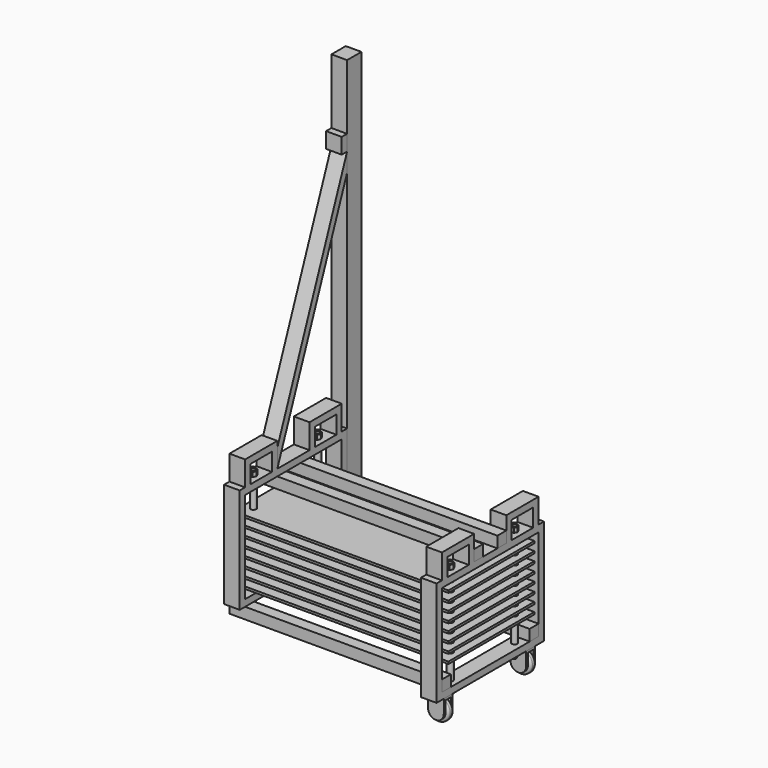
from build123d import *

# Parameters (mm, degrees)
F0_W           = 1219.2
F0_H           = 609.6
F0_R           = 12.7
F1_DEPTH       = 12.7
F9_R           = 15.875
F9_R_2         = 12.7
F10_DEPTH      = 127
F10_DEPTH_BACK = 393.7
F29_DEPTH      = 25.4
F29_DEPTH_BACK = 495.3
F9_R_3         = 9.525
F46_DEPTH      = 203.2
F46_DEPTH_BACK = 469.9
F47_DEPTH      = 101.6
F47_DEPTH_BACK = 571.5
F49_DEPTH      = 88.9
F57_W          = 38.1
F57_H          = 520.7
F58_DEPTH      = 88.9
F59_W          = 38.1
F59_H          = 520.7
F60_DEPTH      = 88.9
F62_DEPTH      = 88.9
F64_DEPTH      = 88.9
F66_DEPTH      = 710.8932972611
F67_R          = 60.325
F68_DEPTH      = 38.1
F69_R          = 12.7
F71_R          = 9.525
F72_DEPTH      = 25.4
F84_DEPTH      = 88.9
F85_W          = 63.5
F85_H          = 63.5
F86_DEPTH      = 1206.5
F88_DEPTH      = 88.9
F90_DEPTH      = 88.9
F89_W          = 38.1
F89_H          = 88.9
F91_DEPTH      = 88.9


with BuildPart() as f1:
    # F0 (on Top) → F1 (new body)
    with BuildSketch(Plane.XY):
        with Locations((1.1357478797, 12.4982790879)):
            Rectangle(F0_W, F0_H)
        with Locations((-557.6642521203, -216.1017209121)):
            Circle(F0_R, mode=Mode.SUBTRACT)
        with Locations((559.9357478797, -216.1017209121)):
            Circle(F0_R, mode=Mode.SUBTRACT)
        with Locations((-557.6642521203, 241.0982790879)):
            Circle(F0_R, mode=Mode.SUBTRACT)
        with Locations((559.9357478797, 241.0982790879)):
            Circle(F0_R, mode=Mode.SUBTRACT)
    extrude(amount=F1_DEPTH)


with BuildPart() as f2_1:
    # F2: copy of F1
    add(f1.part.moved(Location((0, 0, -50.8))))


with BuildPart() as f3_1:
    # F3: copy of F2_1
    add(f2_1.part.moved(Location((0, 0, -50.8))))


with BuildPart() as f4_1:
    # F4: copy of F3_1
    add(f3_1.part.moved(Location((0, 0, -50.8))))


with BuildPart() as f5_1:
    # F5: copy of F4_1
    add(f4_1.part.moved(Location((0, 0, -50.8))))


with BuildPart() as f6_1:
    # F6: copy of F5_1
    add(f5_1.part.moved(Location((0, 0, -50.8))))


with BuildPart() as f7_1:
    # F7: copy of F6_1
    add(f6_1.part.moved(Location((0, 0, -50.8))))


with BuildPart() as f8_1:
    # F8: copy of F7_1
    add(f7_1.part.moved(Location((0, 0, -50.8))))


with BuildPart() as f10:
    # F9 (on face) → F10 (new body, two sides)
    with BuildSketch(Plane.XY.offset(12.7)) as f10_sk:
        with Locations((-557.6642521203, 241.0982790879)):
            Circle(F9_R)
        with Locations((-557.6642521203, 241.0982790879)):
            Circle(F9_R_2, mode=Mode.SUBTRACT)
    extrude(amount=F10_DEPTH)
    extrude(f10_sk.sketch, amount=-F10_DEPTH_BACK)

    # F12: cut F1
    add(f1.part, mode=Mode.SUBTRACT)

    # F14: cut F2_1
    add(f2_1.part, mode=Mode.SUBTRACT)


with BuildPart() as f10b:
    # F9 (on face) → F10, piece 2 (new body, two sides)
    with BuildSketch(Plane.XY.offset(12.7)) as f10_2_sk:
        with Locations((-557.6642521203, -216.1017209121)):
            Circle(F9_R)
        with Locations((-557.6642521203, -216.1017209121)):
            Circle(F9_R_2, mode=Mode.SUBTRACT)
    extrude(amount=F10_DEPTH)
    extrude(f10_2_sk.sketch, amount=-F10_DEPTH_BACK)

    # F12: cut F1
    add(f1.part, mode=Mode.SUBTRACT)

    # F14: cut F2_1
    add(f2_1.part, mode=Mode.SUBTRACT)


with BuildPart() as f11_1:
    # F11: copy of F1
    add(f1.part)


with BuildPart() as f13_1:
    # F13: copy of F2_1
    add(f2_1.part)


with BuildPart() as f15_1:
    # F15: copy of F13_1
    add(f13_1.part)


with BuildPart() as f10_1:
    add(f10.part)

    # F16: cut F13_1
    add(f13_1.part, mode=Mode.SUBTRACT)


with BuildPart() as f10b_1:
    add(f10b.part)

    # F16: cut F13_1
    add(f13_1.part, mode=Mode.SUBTRACT)


with BuildPart() as f17_1:
    # F17: copy of F3_1
    add(f3_1.part)


with BuildPart() as f10_2:
    add(f10_1.part)

    # F18: cut F17_1
    add(f17_1.part, mode=Mode.SUBTRACT)


with BuildPart() as f10b_2:
    add(f10b_1.part)

    # F18: cut F17_1
    add(f17_1.part, mode=Mode.SUBTRACT)


with BuildPart() as f19_1:
    # F19: copy of F4_1
    add(f4_1.part)


with BuildPart() as f10_3:
    add(f10_2.part)

    # F20: cut F19_1
    add(f19_1.part, mode=Mode.SUBTRACT)


with BuildPart() as f10b_3:
    add(f10b_2.part)

    # F20: cut F19_1
    add(f19_1.part, mode=Mode.SUBTRACT)


with BuildPart() as f21_1:
    # F21: copy of F5_1
    add(f5_1.part)


with BuildPart() as f10_4:
    add(f10_3.part)

    # F22: cut F21_1
    add(f21_1.part, mode=Mode.SUBTRACT)


with BuildPart() as f10b_4:
    add(f10b_3.part)

    # F22: cut F21_1
    add(f21_1.part, mode=Mode.SUBTRACT)


with BuildPart() as f23_1:
    # F23: copy of F6_1
    add(f6_1.part)


with BuildPart() as f10_5:
    add(f10_4.part)

    # F24: cut F23_1
    add(f23_1.part, mode=Mode.SUBTRACT)


with BuildPart() as f10b_5:
    add(f10b_4.part)

    # F24: cut F23_1
    add(f23_1.part, mode=Mode.SUBTRACT)


with BuildPart() as f25_1:
    # F25: copy of F7_1
    add(f7_1.part)


with BuildPart() as f10_6:
    add(f10_5.part)

    # F26: cut F25_1
    add(f25_1.part, mode=Mode.SUBTRACT)


with BuildPart() as f10b_6:
    add(f10b_5.part)

    # F26: cut F25_1
    add(f25_1.part, mode=Mode.SUBTRACT)


with BuildPart() as f27_1:
    # F27: copy of F8_1
    add(f8_1.part)


with BuildPart() as f10_7:
    add(f10_6.part)

    # F28: cut F27_1
    add(f27_1.part, mode=Mode.SUBTRACT)


with BuildPart() as f10b_7:
    add(f10b_6.part)

    # F28: cut F27_1
    add(f27_1.part, mode=Mode.SUBTRACT)


with BuildPart() as f29:
    # F9 (on face) → F29 (new body, two sides)
    with BuildSketch(Plane.XY.offset(12.7)) as f29_sk:
        with Locations((559.9357478797, 241.0982790879)):
            Circle(F9_R)
        with Locations((559.9357478797, 241.0982790879)):
            Circle(F9_R_2, mode=Mode.SUBTRACT)
    extrude(amount=F29_DEPTH)
    extrude(f29_sk.sketch, amount=-F29_DEPTH_BACK)

    # F31: cut F11_1
    add(f11_1.part, mode=Mode.SUBTRACT)


with BuildPart() as f29b:
    # F9 (on face) → F29, piece 2 (new body, two sides)
    with BuildSketch(Plane.XY.offset(12.7)) as f29_2_sk:
        with Locations((559.9357478797, -216.1017209121)):
            Circle(F9_R)
        with Locations((559.9357478797, -216.1017209121)):
            Circle(F9_R_2, mode=Mode.SUBTRACT)
    extrude(amount=F29_DEPTH)
    extrude(f29_2_sk.sketch, amount=-F29_DEPTH_BACK)

    # F31: cut F11_1
    add(f11_1.part, mode=Mode.SUBTRACT)


with BuildPart() as f30_1:
    # F30: copy of F11_1
    add(f11_1.part)


with BuildPart() as f32_1:
    # F32: copy of F15_1
    add(f15_1.part)


with BuildPart() as f29_1:
    add(f29.part)

    # F33: cut F32_1
    add(f32_1.part, mode=Mode.SUBTRACT)

    # F35: cut F3_1
    add(f3_1.part, mode=Mode.SUBTRACT)

    # F37: cut F5_1
    add(f5_1.part, mode=Mode.SUBTRACT)

    # F39: cut F4_1
    add(f4_1.part, mode=Mode.SUBTRACT)

    # F41: cut F6_1
    add(f6_1.part, mode=Mode.SUBTRACT)

    # F43: cut F7_1
    add(f7_1.part, mode=Mode.SUBTRACT)

    # F45: cut F8_1
    add(f8_1.part, mode=Mode.SUBTRACT)


with BuildPart() as f29b_1:
    add(f29b.part)

    # F33: cut F32_1
    add(f32_1.part, mode=Mode.SUBTRACT)

    # F35: cut F3_1
    add(f3_1.part, mode=Mode.SUBTRACT)

    # F37: cut F5_1
    add(f5_1.part, mode=Mode.SUBTRACT)

    # F39: cut F4_1
    add(f4_1.part, mode=Mode.SUBTRACT)

    # F41: cut F6_1
    add(f6_1.part, mode=Mode.SUBTRACT)

    # F43: cut F7_1
    add(f7_1.part, mode=Mode.SUBTRACT)

    # F45: cut F8_1
    add(f8_1.part, mode=Mode.SUBTRACT)


with BuildPart() as f34_1:
    # F34: copy of F3_1
    add(f3_1.part)


with BuildPart() as f36_1:
    # F36: copy of F5_1
    add(f5_1.part)


with BuildPart() as f38_1:
    # F38: copy of F4_1
    add(f4_1.part)


with BuildPart() as f40_1:
    # F40: copy of F6_1
    add(f6_1.part)


with BuildPart() as f42_1:
    # F42: copy of F7_1
    add(f7_1.part)


with BuildPart() as f44_1:
    # F44: copy of F8_1
    add(f8_1.part)


with BuildPart() as f46:
    # F9 (on face) → F46 (new body, two sides)
    with BuildSketch(Plane.XY.offset(12.7)) as f46_sk:
        with Locations((-557.6642521203, 241.0982790879)):
            Circle(F9_R_3)
    extrude(amount=F46_DEPTH)
    extrude(f46_sk.sketch, amount=-F46_DEPTH_BACK)


with BuildPart() as f46b:
    # F9 (on face) → F46, piece 2 (new body, two sides)
    with BuildSketch(Plane.XY.offset(12.7)) as f46_2_sk:
        with Locations((-557.6642521203, -216.1017209121)):
            Circle(F9_R_3)
    extrude(amount=F46_DEPTH)
    extrude(f46_2_sk.sketch, amount=-F46_DEPTH_BACK)


with BuildPart() as f47:
    # F9 (on face) → F47 (new body, two sides)
    with BuildSketch(Plane.XY.offset(12.7)) as f47_sk:
        with Locations((559.9357478797, -216.1017209121)):
            Circle(F9_R_3)
    extrude(amount=F47_DEPTH)
    extrude(f47_sk.sketch, amount=-F47_DEPTH_BACK)


with BuildPart() as f47b:
    # F9 (on face) → F47, piece 2 (new body, two sides)
    with BuildSketch(Plane.XY.offset(12.7)) as f47_2_sk:
        with Locations((559.9357478797, 241.0982790879)):
            Circle(F9_R_3)
    extrude(amount=F47_DEPTH)
    extrude(f47_2_sk.sketch, amount=-F47_DEPTH_BACK)


with BuildPart() as f49:
    # F48 (on face) → F49 (new body)
    with BuildSketch(Plane.YZ.offset(610.7357478797)):
        Polygon((-368.5017209121, 38.1), (-292.3017209121, 38.1), (317.2982790879, 38.1), (393.4982790879, 38.1), (393.4982790879, 76.2), (317.2982790879, 76.2), (-292.3017209121, 76.2), (-368.5017209121, 76.2), align=None)
    extrude(amount=F49_DEPTH)


with BuildPart() as f49_1:
    # F50: moved
    add(f49.part.moved(Location((-95.25, 0, 0))))

    # F53: cut F47b, F47
    add(f47b.part, mode=Mode.SUBTRACT)
    add(f47.part, mode=Mode.SUBTRACT)


with BuildPart() as f51_1:
    # F51: copy of F47b
    add(f47b.part)


with BuildPart() as f52_1:
    # F52: copy of F47
    add(f47.part)


with BuildPart() as f54_1:
    # F54: copy of F49
    add(f49_1.part.moved(Location((0, 0, -558.8))))


with BuildPart() as f55_1:
    # F55: copy of F49
    add(f49_1.part.moved(Location((-1117.6, 0, 101.6))))


with BuildPart() as f56_1:
    # F56: copy of F55_1
    add(f55_1.part.moved(Location((0, 0, -558.8))))


with BuildPart() as f49_2:
    add(f49_1.part)

    add(f54_1.part)  # F58 merges F54_1
    # F57 (on face) → F58 (join, through all)
    with BuildSketch(Plane.YZ.offset(604.3857478797)):
        with Locations((-349.4517209121, -222.25)):
            Rectangle(F57_W, F57_H)
        with Locations((374.4482790879, -222.25)):
            Rectangle(F57_W, F57_H)
    extrude(amount=-F58_DEPTH)

    # F83 (on face) → F84 (join, through all)
    with BuildSketch(Plane.YZ.offset(604.3857478797)):
        Polygon((126.7982790879, 215.9), (126.7982790879, 76.2), (164.8982790879, 76.2), (164.8982790879, 177.8), (317.2982790879, 177.8), (317.2982790879, 76.2), (355.3982790879, 76.2), (355.3982790879, 215.9), align=None)
        Polygon((-330.4017209121, 215.9), (-330.4017209121, 76.2), (-292.3017209121, 76.2), (-292.3017209121, 177.8), (-139.9017209121, 177.8), (-139.9017209121, 76.2), (-101.8017209121, 76.2), (-101.8017209121, 215.9), align=None)
    extrude(amount=-F84_DEPTH)


with BuildPart() as f55_1_1:
    add(f55_1.part)

    add(f56_1.part)  # F60 merges F56_1
    # F59 (on face) → F60 (join, through all)
    with BuildSketch(Plane(origin=(-602.1142521203, 0, 0), x_dir=(0, -1, 0), z_dir=(-1, 0, 0))):
        with Locations((349.4517209121, -120.65)):
            Rectangle(F59_W, F59_H)
        with Locations((-374.4482790879, -120.65)):
            Rectangle(F59_W, F59_H)
    extrude(amount=-F60_DEPTH)

    # F61 (on face) → F62 (join, through all)
    with BuildSketch(Plane(origin=(-602.1142521203, 0, 0), x_dir=(0, -1, 0), z_dir=(-1, 0, 0))):
        Polygon((-355.3982790879, 317.5), (-355.3982790879, 177.8), (-317.2982790879, 177.8), (-317.2982790879, 279.4), (-164.8982790879, 279.4), (-164.8982790879, 177.8), (-126.7982790879, 177.8), (-126.7982790879, 317.5), align=None)
        Polygon((292.3017209121, 177.8), (330.4017209121, 177.8), (330.4017209121, 317.5), (101.8017209121, 317.5), (101.8017209121, 177.8), (139.9017209121, 177.8), (139.9017209121, 279.4), (292.3017209121, 279.4), align=None)
    extrude(amount=-F62_DEPTH)


with BuildPart() as f64:
    # F63 (on face) → F64 (new body, through all)
    with BuildSketch(Plane.YZ.offset(604.3857478797)):
        Polygon((-253.8940181732, -520.7), (-317.3940181732, -520.7), (-317.3940181732, -673.1), (-304.6940181732, -673.1), (-304.6940181732, -533.4), (-266.5940181732, -533.4), (-266.5940181732, -673.1), (-253.8940181732, -673.1), align=None)
    extrude(amount=-F64_DEPTH)


with BuildPart() as f64b:
    # F63 (on face) → F64, piece 2 (new body, through all)
    with BuildSketch(Plane.YZ.offset(604.3857478797)):
        Polygon((330.6414017677, -673.1), (330.6414017677, -520.7), (267.1414017677, -520.7), (267.1414017677, -673.1), (279.8414017677, -673.1), (279.8414017677, -533.4), (317.9414017677, -533.4), (317.9414017677, -673.1), align=None)
    extrude(amount=-F64_DEPTH)


with BuildPart() as f66_tool:
    # F65 (on face) → F66 (new body, through all)
    with BuildSketch(Plane.XZ.offset(317.3940181732)):
        with BuildLine():
            ThreePointArc((604.3857478797, -596.9), (559.9357478797, -641.35), (515.4857478797, -596.9))
            Line((515.4857478797, -596.9), (515.4857478797, -673.1))
            Line((515.4857478797, -673.1), (604.3857478797, -673.1))
            Line((604.3857478797, -673.1), (604.3857478797, -596.9))
        make_face()
    extrude(amount=-F66_DEPTH)


with BuildPart() as f64_1:
    add(f64.part)

    # F66: cut by f66_tool
    add(f66_tool.part, mode=Mode.SUBTRACT)


with BuildPart() as f64b_1:
    add(f64b.part)

    # F66: cut by f66_tool
    add(f66_tool.part, mode=Mode.SUBTRACT)


with BuildPart() as f68:
    # F67 (on face) → F68 (new body, through all)
    with BuildSketch(Plane.XZ.offset(266.5940181732)):
        with Locations((559.9357478797, -596.9)):
            Circle(F67_R)
    extrude(amount=F68_DEPTH)

    # F69
    f69_edges = [f68.edges().sort_by_distance(p)[0] for p in [
        (620.260748, -285.644018, -596.9),
        (499.610748, -266.594018, -596.9),
        (499.610748, -304.694018, -596.9),
    ]]
    fillet(f69_edges, radius=F69_R)


with BuildPart() as f70_1:
    # F70: copy of F68
    add(f68.part.moved(Location((0, 584.5018, 0))))


with BuildPart() as f72:
    # F71 (on face) → F72 (new body)
    with BuildSketch(Plane.XY.offset(177.8)):
        Polygon((-567.1892521203, 258.4611697068), (-575.0271427392, 241.0982790879), (-567.1892521203, 223.7353884689), (-548.1392521203, 223.7353884689), (-540.3013615013, 241.0982790879), (-548.1392521203, 258.4611697068), align=None)
        with Locations((-557.6642521203, 241.0982790879)):
            Circle(F71_R, mode=Mode.SUBTRACT)
    extrude(amount=F72_DEPTH)


with BuildPart() as f72b:
    # F71 (on face) → F72, piece 2 (new body)
    with BuildSketch(Plane.XY.offset(177.8)):
        Polygon((-567.1892521203, -198.7388302932), (-575.0271427392, -216.1017209121), (-567.1892521203, -233.4646115311), (-548.1392521203, -233.4646115311), (-540.3013615013, -216.1017209121), (-548.1392521203, -198.7388302932), align=None)
        with Locations((-557.6642521203, -216.1017209121)):
            Circle(F71_R, mode=Mode.SUBTRACT)
    extrude(amount=F72_DEPTH)


with BuildPart() as f73_1:
    # F73: copy of F72
    add(f72.part.moved(Location((0, 0, -622.3))))

    # F75: cut F46
    add(f46.part, mode=Mode.SUBTRACT)


with BuildPart() as f74_1:
    # F74: copy of F46
    add(f46.part)


with BuildPart() as f72_1:
    add(f72.part)

    # F75: cut F46
    add(f46.part, mode=Mode.SUBTRACT)


with BuildPart() as f76_1:
    # F76: copy of F72b
    add(f72b.part.moved(Location((0, 0, -622.3))))

    # F78: cut F46b
    add(f46b.part, mode=Mode.SUBTRACT)


with BuildPart() as f77_1:
    # F77: copy of F46b
    add(f46b.part)


with BuildPart() as f72b_1:
    add(f72b.part)

    # F78: cut F46b
    add(f46b.part, mode=Mode.SUBTRACT)


with BuildPart() as f79_1:
    # F79: copy of F72b
    add(f72b_1.part.moved(Location((1117.6, 0, -101.6))))


with BuildPart() as f80_1:
    # F80: copy of F79_1
    add(f79_1.part.moved(Location((0, 457.2, 0))))


with BuildPart() as f81_1:
    # F81: copy of F79_1
    add(f79_1.part.moved(Location((0, 0, -622.3))))


with BuildPart() as f82_1:
    # F82: copy of F80_1
    add(f80_1.part.moved(Location((0, 0, -622.3))))


with BuildPart() as f86:
    # F85 (on face) → F86 (new body, through all)
    with BuildSketch(Plane.YZ.offset(604.3857478797)):
        with Locations((-298.6517209121, -450.85)):
            Rectangle(F85_W, F85_H)
    extrude(amount=-F86_DEPTH)


with BuildPart() as f86b:
    # F85 (on face) → F86, piece 2 (new body, through all)
    with BuildSketch(Plane.YZ.offset(604.3857478797)):
        with Locations((323.6482790879, -450.85)):
            Rectangle(F85_W, F85_H)
    extrude(amount=-F86_DEPTH)


with BuildPart() as f86c:
    # F85 (on face) → F86, piece 3 (new body, through all)
    with BuildSketch(Plane.YZ.offset(604.3857478797)):
        with Locations((-70.0517209121, 107.95)):
            Rectangle(F85_W, F85_H)
    extrude(amount=-F86_DEPTH)


with BuildPart() as f86d:
    # F85 (on face) → F86, piece 4 (new body, through all)
    with BuildSketch(Plane.YZ.offset(604.3857478797)):
        with Locations((95.0482790879, 107.95)):
            Rectangle(F85_W, F85_H)
    extrude(amount=-F86_DEPTH)


with BuildPart() as f88:
    # F87 (on face) → F88 (new body, through all)
    with BuildSketch(Plane.YZ.offset(-513.2142521203)):
        Polygon((-101.8017209121, 283.2905607781), (-101.8017209121, 177.8), (393.4982790879, 1456.6094392219), (393.4982790879, 1562.1), align=None)
    extrude(amount=-F88_DEPTH)


with BuildPart() as f90:
    # F89 (on face) → F90 (new body, through all)
    with BuildSketch(Plane.YZ.offset(-513.2142521203)):
        Polygon((393.4982790879, 177.8), (393.4982790879, -419.1), (495.0982790879, -419.1), (495.0982790879, 2019.3), (393.4982790879, 2019.3), (393.4982790879, 1651), (393.4982790879, 1562.1), align=None)
    extrude(amount=-F90_DEPTH)


with BuildPart() as f91:
    # F89 (on face) → F91 (new body, through all)
    with BuildSketch(Plane.YZ.offset(-513.2142521203)):
        with Locations((374.4482790879, 1606.55)):
            Rectangle(F89_W, F89_H)
    extrude(amount=-F91_DEPTH)


solid = Compound([f15_1.part, f10_7.part, f10b_7.part, f30_1.part, f29_1.part, f29b_1.part, f34_1.part, f36_1.part, f38_1.part, f40_1.part, f42_1.part, f44_1.part, f51_1.part, f52_1.part, f49_2.part, f55_1_1.part, f64_1.part, f64b_1.part, f68.part, f70_1.part, f73_1.part, f74_1.part, f72_1.part, f76_1.part, f77_1.part, f72b_1.part, f79_1.part, f80_1.part, f81_1.part, f82_1.part, f86.part, f86b.part, f86c.part, f86d.part, f88.part, f90.part, f91.part])
